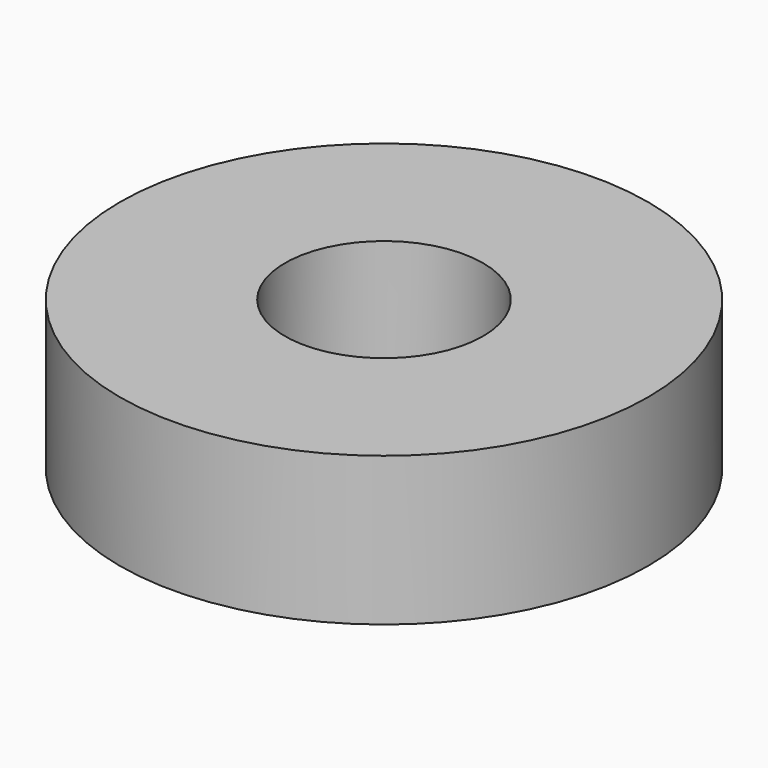
from build123d import *

# Parameters (mm, degrees)
F0_R     = 25.4
F0_R_2   = 9.525
F1_DEPTH = 14.2875


# Not quite as in the source:
# - a length typed as a fraction of an inch, garbled in the dataset ("3 / 203.2 mm" for 3/8 in), is restored


with BuildPart() as f1:
    # F0 (on Top) → F1 (new body)
    with BuildSketch(Plane.XY):
        Circle(F0_R)
        Circle(F0_R_2, mode=Mode.SUBTRACT)
    extrude(amount=F1_DEPTH)


solid = f1.part
